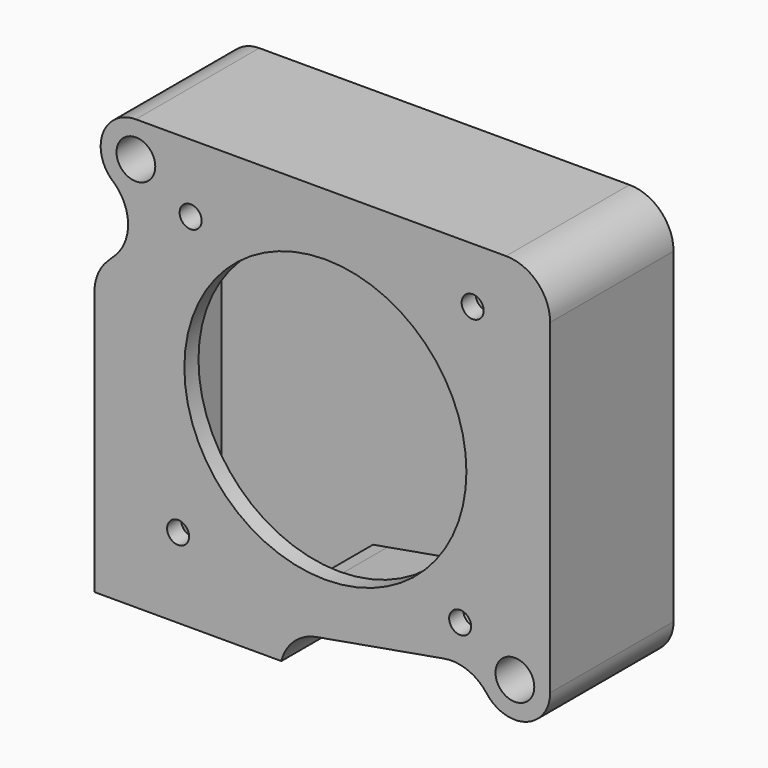
from build123d import *

# Parameters (mm, degrees)
F0_R        = 2.2
F1_DEPTH    = 17.5
F3_DEPTH    = 17.5
F4_T        = 2
F4_T3_DEPTH = 21.5
F5_T1_DEPTH = 17.5
F5_T3_DEPTH = 17.5
F5_T5_DEPTH = 17.5
F5_T7_DEPTH = 42.5
F5_T9_DEPTH = 27.8553390593
F7_D        = 32
F7_DEPTH    = 4
F7_TIP      = 9.6137699044
F8_D        = 2.5
F8_DEPTH    = 4
F8_TIP      = 0.7510757738


# Not quite as in the source:
# - a fillet or chamfer that OpenCascade refuses, or shapes differently, is made with other operations: its cross-section is extruded or revolved along the edge and cut away or added
# - a shell that OpenCascade refuses in one call is made with other operations: the cavity is built on its own and cut out


with BuildPart() as f1:
    # F0 (on Front) → F1 (new body)
    with BuildSketch(Plane.XZ):
        with BuildLine():
            Line((25.5, -19), (25.5, 23))
            Line((25.5, 23), (-21.5, 23))
            ThreePointArc((-21.5, 23), (-25.5, 19), (-21.5, 15))
            Line((-21.5, 15), (17.5, 15))
            Line((17.5, 15), (17.5, -19))
            ThreePointArc((17.5, -19), (21.5, -23), (25.5, -19))
        make_face()
        with Locations((21.5, -19)):
            Circle(F0_R, mode=Mode.SUBTRACT)
        with Locations((-21.5, 19)):
            Circle(F0_R, mode=Mode.SUBTRACT)
    extrude(amount=F1_DEPTH)

    # F2 (on Front) → F3 (join, through all)
    with BuildSketch(Plane.XZ):
        Polygon((17.5, -18.7826429341), (17.5, 15), (-17.5, 15), (-26.2, 6.3), (-26.2, -25.75), (-5, -25.75), (-5, -22.75), align=None)
    extrude(amount=F3_DEPTH)

    # F4: shell of thickness 2, made by hand


with BuildPart() as f4_core1:
    # F4_t2: copy of F1
    add(f1.part)

    # the walls: a layer under each face that stays
    f4_faces = [f4_core1.faces().sort_by_distance(p)[0] for p in [
        (25.5, -8.75, 2),
        (21.5, -8.75, -23),
        (2, -8.75, 23),
        (-0.35, 0, -1.375),
        (-0.35, -17.5, -1.375),
        (17.5, -8.75, -18.891321467),
        (-25.5, -8.75, 19),
        (-19.5, -8.75, 15),
        (19.3, -8.75, -19),
        (-23.7, -8.75, 19),
        (6.25, -8.75, -20.766321467),
        (-21.85, -8.75, 10.65),
        (-26.2, -8.75, -9.725),
        (-5, -8.75, -24.25),
    ]]
    thicken(f4_faces, amount=-F4_T, mode=Mode.SUBTRACT)

    # F4_s4 → F4_t3 (cut)
    with BuildSketch(Plane.XZ.offset(-2)):
        Polygon((17.4834729636, -18.8023390891), (19.5, -18.7826429341), (19.5, -16.3991357489), (17.1527036447, -16.813027428), align=None)
        Polygon((-17.5141421356, 14.9941421356), (-17.5, 17), (-12.6715728753, 17), (-16.0857864376, 13.5857864376), align=None)
        Polygon((-4.9765270364, -22.7696961551), (-5.3472963553, -20.780384494), (-7, -21.0718007376), (-7, -22.75), align=None)
    extrude(amount=F4_T3_DEPTH, mode=Mode.SUBTRACT)


with BuildPart() as f1_1:
    add(f1.part)

    # what is left inside the walls is the cavity
    f4_cavity = [f4_core1.part.solids().sort_by_distance(p)[0] for p in [
        (-0.35, -15.48, -10.166667),
    ]]
    add(f4_cavity, mode=Mode.SUBTRACT)

    # F5: fillet of radius 5 on 5 edges, made by hand

    # F5_s2 → F5_t1 (join)
    with BuildSketch(Plane.XZ):
        with BuildLine():
            ThreePointArc((18.307091383, -21.4094261897), (16.1468840352, -19.7684999194), (13.4477147235, -19.4971701618))
            Line((13.4477147235, -19.4971701618), (13.3608906347, -19.0047662853))
            Line((13.3608906347, -19.0047662853), (17.4131759112, -18.2902390576))
            Line((17.4131759112, -18.2902390576), (18, -18.7826429341))
            ThreePointArc((18, -18.7826429341), (18, -19), (18.7062049602, -21.108247916))
            Line((18.7062049602, -21.108247916), (18.307091383, -21.4094261897))
        make_face()
    extrude(amount=F5_T1_DEPTH)

    # F5_s4 → F5_t3 (join)
    with BuildSketch(Plane.XZ):
        with BuildLine():
            ThreePointArc((-23.8469891482, 8.6530108518), (-22.3858577587, 12.3711260424), (-24.1144546907, 15.972686559))
            Line((-24.1144546907, 15.972686559), (-23.7876478544, 16.3511007391))
            ThreePointArc((-23.7876478544, 16.3511007391), (-21.5, 15.5), (-17.5, 15.5))
            Line((-17.5, 15.5), (-17.1464466094, 14.6464466094))
            Line((-17.1464466094, 14.6464466094), (-23.4934357576, 8.2994574612))
            Line((-23.4934357576, 8.2994574612), (-23.8469891482, 8.6530108518))
        make_face()
    extrude(amount=F5_T3_DEPTH)

    # F5_s6 → F5_t5 (join)
    with BuildSketch(Plane.XZ):
        with BuildLine():
            ThreePointArc((-1.0199301517, -22.0482063006), (-3.5569146257, -23.311037583), (-5, -25.75))
            Line((-5, -25.75), (-5, -22.75))
            Line((-5, -22.75), (-1.0199301517, -22.0482063006))
        make_face()
    extrude(amount=F5_T5_DEPTH)

    # F5_s8 → F5_t7 (cut)
    with BuildSketch(Plane.XZ.offset(-12.5)):
        with BuildLine():
            ThreePointArc((25.5, 18), (24.0355339059, 21.5355339059), (20.5, 23))
            Line((20.5, 23), (25.5, 23))
            Line((25.5, 23), (25.5, 18))
        make_face()
    extrude(amount=F5_T7_DEPTH, mode=Mode.SUBTRACT)

    # F5_s10 → F5_t9 (cut)
    with BuildSketch(Plane.XZ.offset(-5.1776695297)):
        with BuildLine():
            ThreePointArc((-26.2, 4.2289321881), (-25.8193976626, 6.14234935), (-24.7355339059, 7.7644660941))
            Line((-24.7355339059, 7.7644660941), (-26.2, 6.3))
            Line((-26.2, 6.3), (-26.2, 4.2289321881))
        make_face()
    extrude(amount=F5_T9_DEPTH, mode=Mode.SUBTRACT)

    # F7
    with Locations(Plane.XZ.offset(17.5)):
        with Locations((0, 0)):
            Hole(F7_D / 2, depth=F7_DEPTH)
            with Locations((0, 0, -(F7_DEPTH + F7_TIP / 2))):  # 118° drill point
                Cone(0, F7_D / 2, F7_TIP, mode=Mode.SUBTRACT)

    # F8
    with Locations(Plane.XZ.offset(17.5)):
        with Locations((-15.2900823734, 15.2900823734), (-16.7099176266, -16.7099176266), (15.2900823734, -15.2900823734), (16.7099176266, 16.7099176266)):
            Hole(F8_D / 2, depth=F8_DEPTH)
            with Locations((0, 0, -(F8_DEPTH + F8_TIP / 2))):  # 118° drill point
                Cone(0, F8_D / 2, F8_TIP, mode=Mode.SUBTRACT)


solid = f1_1.part
